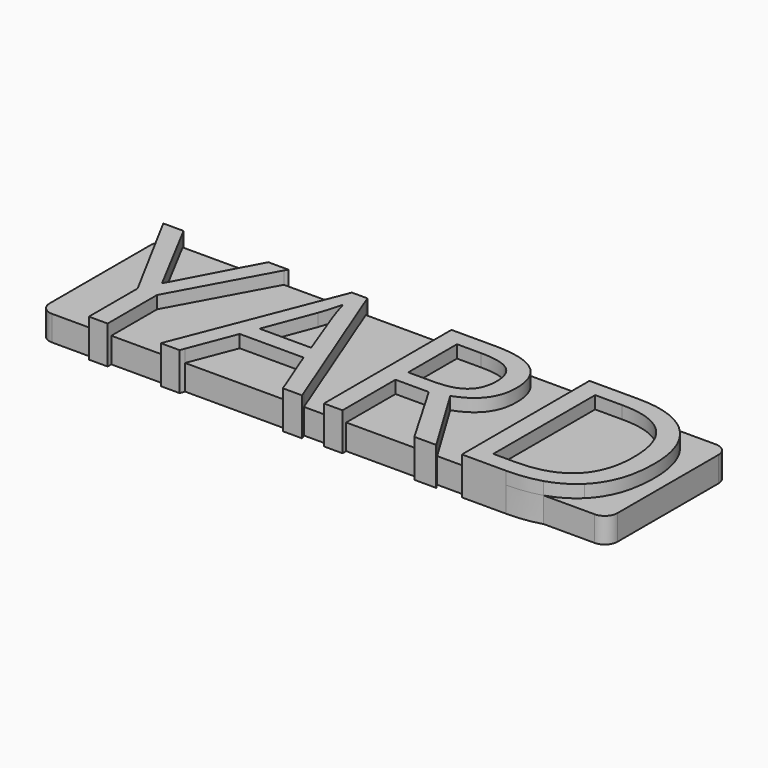
from build123d import *

# Parameters (mm, degrees)
F0_W          = 90
F0_H          = 24
F1_DEPTH      = 4
F2_R          = 2
F3_W          = 2.9686732187
F3_H          = 0.7371007371
F3_W_2        = 2.9355036855
F4_DEPTH      = 2
F4_DEPTH_BACK = 4
F5_TEXT_SIZE  = 17.3611111111
F6_DEPTH      = 1.5


# Not quite as in the source:
# - a feature names something its author has since deleted; it is built from what else it names
# - Text() gives the source's letters only with a copy of the font that has no kerning and outlines rounded to 1/6400 em; it was checked with that copy


with BuildPart() as f1:
    # F0 (on Top) → F1 (new body)
    with BuildSketch(Plane.XY):
        Rectangle(F0_W, F0_H)
    extrude(amount=F1_DEPTH)

    # F2
    f2_edges = [f1.edges().sort_by_distance(p)[0] for p in [
        (-45, -12, 2),
        (45, 12, 2),
        (-45, 12, 2),
        (45, -12, 2),
    ]]
    fillet(f2_edges, radius=F2_R)

    # F3 (on face) → F4 (join, two sides)
    with BuildSketch(Plane.XY.offset(4)) as f4_sk:
        with BuildLine():
            Line((-28.6434596423, 12), (-35.0988943489, -0.1105651106))
            Line((-35.0988943489, -0.1105651106), (-41.5119288276, 12))
            Line((-41.5119288276, 12), (-43, 12))
            ThreePointArc((-43, 12), (-43.760525738, 11.8497569034), (-44.4067877341, 11.4216006018))
            Line((-44.4067877341, 11.4216006018), (-36.585995086, -3.0792383292))
            Line((-36.585995086, -3.0792383292), (-36.585995086, -12))
            Line((-36.585995086, -12), (-33.6173218673, -12))
            Line((-33.6173218673, -12), (-33.6173218673, -2.941031941))
            Line((-33.6173218673, -2.941031941), (-25.4710674125, 12))
            Line((-25.4710674125, 12), (-28.6434596423, 12))
        make_face()
        Polygon((-28.3654791155, 12.5214987715), (-28.6434596423, 12), (-25.4710674125, 12), (-25.1867321867, 12.5214987715), align=None)
        with BuildLine():
            Line((-43, 12), (-41.5119288276, 12))
            Line((-41.5119288276, 12), (-41.7880835381, 12.5214987715))
            Line((-41.7880835381, 12.5214987715), (-45, 12.5214987715))
            Line((-45, 12.5214987715), (-44.4067877341, 11.4216006018))
            ThreePointArc((-44.4067877341, 11.4216006018), (-43.760525738, 11.8497569034), (-43, 12))
        make_face()
        Polygon((-12.4861748092, 12), (-15.4493294118, 12), (-24.8965831172, -12), (-21.9274304963, -12), (-19.1056511057, -4.7045454545), (-8.9834152334, -4.7045454545), (-6.1264891244, -12), (-3.0860004413, -12), align=None)
        with BuildLine():
            Line((-12.8366093366, 5.765970516), (-9.8955773956, -2.062039312))
            Line((-9.8955773956, -2.062039312), (-18.0663390663, -2.062039312))
            Line((-18.0663390663, -2.062039312), (-15.0976658477, 5.765970516))
            add(Edge.make_bspline(
                [(-14.0085995086, 9.4090909091), (-14.39004914, 7.7506142506), (-15.0976658477, 5.765970516)],
                knots=[0, 0, 0, 1, 1, 1], degree=2))
            add(Edge.make_bspline(
                [(-12.8366093366, 5.765970516), (-13.406019656, 7.2530712531), (-14.0085995086, 9.4090909091)],
                knots=[0, 0, 0, 1, 1, 1], degree=2))
        make_face(mode=Mode.SUBTRACT)
        Polygon((-15.2027027027, 12.6265356265), (-15.4493294118, 12), (-12.4861748092, 12), (-12.7315724816, 12.6265356265), align=None)
        with Locations((-35.1016584767, -12.3685503686)):
            Rectangle(F3_W, F3_H)
        Polygon((-21.9274304963, -12), (-24.8965831172, -12), (-25.1867321867, -12.7371007371), (-22.2125307125, -12.7371007371), align=None)
        Polygon((-2.7972972973, -12.7371007371), (-3.0860004413, -12), (-6.1264891244, -12), (-5.8378378378, -12.7371007371), align=None)
        with BuildLine():
            Line((11.9224593709, 12), (0.6744471744, 12))
            Line((0.6744471744, 12), (0.6744471744, -12))
            Line((0.6744471744, -12), (3.60995086, -12))
            Line((3.60995086, -12), (3.60995086, -2.2334152334))
            Line((3.60995086, -2.2334152334), (8.8839066339, -2.2334152334))
            Line((8.8839066339, -2.2334152334), (14.5690870296, -12))
            Line((14.5690870296, -12), (18.0243381472, -12))
            Line((18.0243381472, -12), (11.6093366093, -1.3875921376))
            add(Edge.make_bspline(
                [(16.6898034398, 5.3845208845), (16.6898034398, 0.3759213759), (11.6093366093, -1.3875921376)],
                knots=[0, 0, 0, 1, 1, 1], degree=2))
            add(Edge.make_bspline(
                [(14.4702088452, 10.7414004914), (16.6898034398, 8.9613022113), (16.6898034398, 5.3845208845)],
                knots=[0, 0, 0, 1, 1, 1], degree=2))
            add(Edge.make_bspline(
                [(11.9224593709, 12), (13.4519884838, 11.5580056131), (14.4702088452, 10.7414004914)],
                knots=[0.5412584064, 0.5412584064, 0.5412584064, 1, 1, 1], degree=2))
        make_face()
        with BuildLine():
            Line((7.64004914, 0.2874692875), (3.60995086, 0.2874692875))
            Line((3.60995086, 0.2874692875), (3.60995086, 9.9453316953))
            Line((3.60995086, 9.9453316953), (7.42997543, 9.9453316953))
            add(Edge.make_bspline(
                [(12.1732186732, 8.8396805897), (10.6971744472, 9.9453316953), (7.42997543, 9.9453316953)],
                knots=[0, 0, 0, 1, 1, 1], degree=2))
            add(Edge.make_bspline(
                [(13.6492628993, 5.2297297297), (13.6492628993, 7.734029484), (12.1732186732, 8.8396805897)],
                knots=[0, 0, 0, 1, 1, 1], degree=2))
            add(Edge.make_bspline(
                [(12.1980958231, 1.523034398), (13.6492628993, 2.7585995086), (13.6492628993, 5.2297297297)],
                knots=[0, 0, 0, 1, 1, 1], degree=2))
            add(Edge.make_bspline(
                [(7.64004914, 0.2874692875), (10.7469287469, 0.2874692875), (12.1980958231, 1.523034398)],
                knots=[0, 0, 0, 1, 1, 1], degree=2))
        make_face(mode=Mode.SUBTRACT)
        with BuildLine():
            Line((0.6744471744, 12.5214987715), (0.6744471744, 12))
            Line((0.6744471744, 12), (11.9224593709, 12))
            add(Edge.make_bspline(
                [(7.6013513514, 12.5214987715), (10.1178039793, 12.5214987715), (11.9224593709, 12)],
                knots=[0, 0, 0, 0.5412584064, 0.5412584064, 0.5412584064], degree=2))
            Line((7.6013513514, 12.5214987715), (0.6744471744, 12.5214987715))
        make_face()
        with Locations((2.1421990172, -12.3685503686)):
            Rectangle(F3_W_2, F3_H)
        with BuildLine():
            Line((34.5746826116, 12), (22.5442260442, 12))
            Line((22.5442260442, 12), (22.5442260442, -12))
            Line((22.5442260442, -12), (34.896240823, -12))
            add(Edge.make_bspline(
                [(39.3114250614, -9.4284398034), (37.5191914784, -11.1754297048), (34.896240823, -12)],
                knots=[0, 0, 0, 0.5280051164, 0.5280051164, 0.5280051164], degree=2))
            add(Edge.make_bspline(
                [(42.7057739558, 0.1326781327), (42.7057739558, -6.1197788698), (39.3114250614, -9.4284398034)],
                knots=[0, 0, 0, 1, 1, 1], degree=2))
            add(Edge.make_bspline(
                [(39.4413390663, 9.2570638821), (42.7057739558, 5.9926289926), (42.7057739558, 0.1326781327)],
                knots=[0, 0, 0, 1, 1, 1], degree=2))
            add(Edge.make_bspline(
                [(34.5746826116, 12), (37.4816642255, 11.2167387229), (39.4413390663, 9.2570638821)],
                knots=[0.3996894081, 0.3996894081, 0.3996894081, 1, 1, 1], degree=2))
        make_face()
        with BuildLine():
            add(Edge.make_bspline(
                [(39.5988943489, 0.0276412776), (39.5988943489, 4.9699017199), (37.1194717445, 7.4742014742)],
                knots=[0, 0, 0, 1, 1, 1], degree=2))
            add(Edge.make_bspline(
                [(36.9536240786, -7.6151719902), (39.5988943489, -5.0307125307), (39.5988943489, 0.0276412776)],
                knots=[0, 0, 0, 1, 1, 1], degree=2))
            add(Edge.make_bspline(
                [(29.0565110565, -10.1996314496), (34.3083538084, -10.1996314496), (36.9536240786, -7.6151719902)],
                knots=[0, 0, 0, 1, 1, 1], degree=2))
            Line((29.0565110565, -10.1996314496), (25.4797297297, -10.1996314496))
            Line((25.4797297297, -10.1996314496), (25.4797297297, 9.9785012285))
            Line((25.4797297297, 9.9785012285), (29.7475429975, 9.9785012285))
            add(Edge.make_bspline(
                [(37.1194717445, 7.4742014742), (34.64004914, 9.9785012285), (29.7475429975, 9.9785012285)],
                knots=[0, 0, 0, 1, 1, 1], degree=2))
        make_face(mode=Mode.SUBTRACT)
        with BuildLine():
            Line((22.5442260442, 12.5214987715), (22.5442260442, 12))
            Line((22.5442260442, 12), (34.5746826116, 12))
            add(Edge.make_bspline(
                [(30.2837837838, 12.5214987715), (32.6392015854, 12.5214987715), (34.5746826116, 12)],
                knots=[0, 0, 0, 0.3996894081, 0.3996894081, 0.3996894081], degree=2))
            Line((30.2837837838, 12.5214987715), (22.5442260442, 12.5214987715))
        make_face()
        Polygon((18.0243381472, -12), (14.5690870296, -12), (14.9981572482, -12.7371007371), (18.4699017199, -12.7371007371), align=None)
        with BuildLine():
            Line((34.896240823, -12), (22.5442260442, -12))
            Line((22.5442260442, -12), (22.5442260442, -12.7371007371))
            Line((22.5442260442, -12.7371007371), (29.542997543, -12.7371007371))
            add(Edge.make_bspline(
                [(34.896240823, -12), (32.5515300412, -12.7371007371), (29.542997543, -12.7371007371)],
                knots=[0.5280051164, 0.5280051164, 0.5280051164, 1, 1, 1], degree=2))
        make_face()
    extrude(amount=F4_DEPTH)
    extrude(f4_sk.sketch, amount=-F4_DEPTH_BACK)

    # F5 (on face) → F6 (cut)
    with BuildSketch(Plane(origin=(0, 0, 0), x_dir=(1, 0, 0), z_dir=(0, 0, -1))):
        with Locations((-23.346625434, -6.25)):
            Text('3 feet', F5_TEXT_SIZE, font='Open Sans', text_align=(TextAlign.LEFT, TextAlign.BOTTOM))
    extrude(amount=-F6_DEPTH, mode=Mode.SUBTRACT)


solid = f1.part
